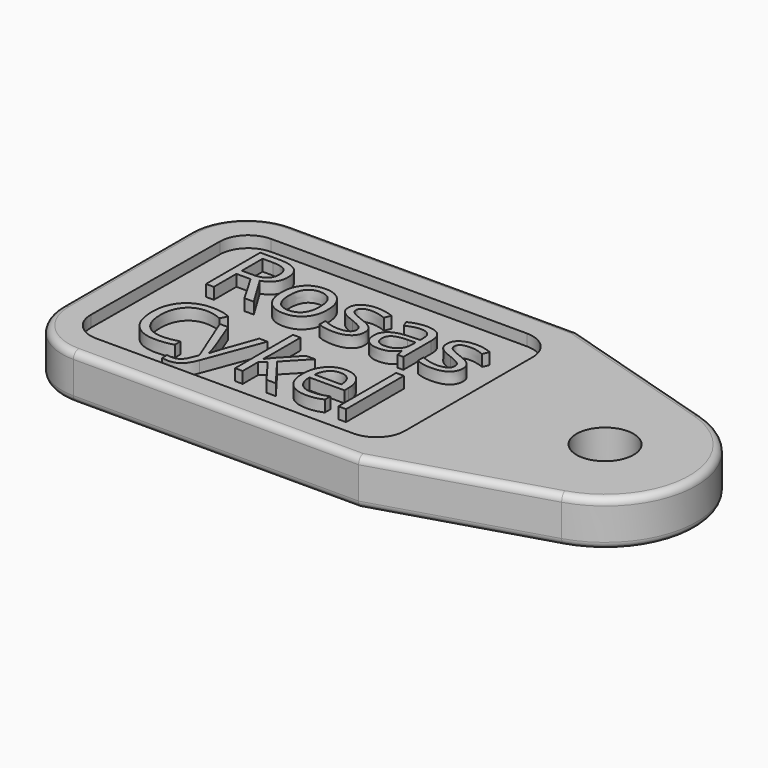
from build123d import *

# Parameters (mm, degrees)
F1_DEPTH     = 3
F2_TEXT_SIZE = 8.3333333333
F3_DEPTH     = 1
F4_R         = 0.6
F5_DEPTH     = 1
F6_D         = 5
F7_R         = 0.6


# Not quite as in the source:
# - Text() gives the source's letters only with a copy of the font that has no kerning and outlines rounded to 1/6400 em; it was checked with that copy


with BuildPart() as f1:
    # F0 (on Top) → F1 (new body)
    with BuildSketch(Plane.XY):
        with BuildLine():
            Line((30, 12), (5, 12))
            ThreePointArc((5, 12), (1.4644660941, 10.5355339059), (0, 7))
            Line((0, 7), (0, -7))
            ThreePointArc((0, -7), (1.4644660941, -10.5355339059), (5, -12))
            Line((5, -12), (30, -12))
            Line((30, -12), (44.322209849, -7.6555431824))
            ThreePointArc((44.322209849, -7.6555431824), (50, 0), (44.322209849, 7.6555431824))
            Line((44.322209849, 7.6555431824), (30, 12))
        make_face()
    extrude(amount=F1_DEPTH)

    # F2 (on face) → F3 (join)
    with BuildSketch(Plane.XY.offset(3)):
        with Locations((5, 1.5)):
            Text('Rosas', F2_TEXT_SIZE, font='Open Sans', text_align=(TextAlign.LEFT, TextAlign.BOTTOM))
        with Locations((5, -7)):
            Text('Cykel', F2_TEXT_SIZE, font='Open Sans', text_align=(TextAlign.LEFT, TextAlign.BOTTOM))
    extrude(amount=F3_DEPTH)

    # F4
    f4_edges = [f1.edges().sort_by_distance(p)[0] for p in [
        (1.464466, -10.535534, 0),
        (37.161105, -9.827772, 0),
    ]]
    fillet(f4_edges, radius=F4_R)

    # F2 (on face) → F5 (join)
    with BuildSketch(Plane.XY.offset(3)):
        with BuildLine():
            ThreePointArc((44.322209849, -7.6555431824), (50, 0), (44.322209849, 7.6555431824))
            Line((44.322209849, 7.6555431824), (30, 12))
            Line((30, 12), (5, 12))
            ThreePointArc((5, 12), (1.4644660941, 10.5355339059), (0, 7))
            Line((0, 7), (0, -7))
            ThreePointArc((0, -7), (1.4644660941, -10.5355339059), (5, -12))
            Line((5, -12), (30, -12))
            Line((30, -12), (44.322209849, -7.6555431824))
        make_face()
        with BuildLine():
            ThreePointArc((2.6266098272, 7.0191604938), (3.3655567355, 8.7745282802), (5.1265364012, 9.5))
            Line((5.1265364012, 9.5), (27.5572421402, 9.5))
            ThreePointArc((27.5572421402, 9.5), (29.3250090931, 8.767766953), (30.0572421402, 7))
            Line((30.0572421402, 7), (30.0572421402, -7))
            ThreePointArc((30.0572421402, -7), (29.3250090931, -8.767766953), (27.5572421402, -9.5))
            Line((27.5572421402, -9.5), (5.0192344847, -9.5))
            ThreePointArc((5.0192344847, -9.5), (3.2447062045, -8.7609796656), (2.5193079106, -6.9808395062))
            Line((2.5193079106, -6.9808395062), (2.6266098272, 7.0191604938))
        make_face(mode=Mode.SUBTRACT)
    extrude(amount=F5_DEPTH)

    # F6 (through all)
    with Locations(Plane(origin=(0, 0, 0), x_dir=(1, 0, 0), z_dir=(0, 0, -1))):
        with Locations((42, 0)):
            Hole(F6_D / 2)

    # F7
    f7_edges = [f1.edges().sort_by_distance(p)[0] for p in [
        (17.5, 12, 4),
        (37.161105, 9.827772, 4),
    ]]
    fillet(f7_edges, radius=F7_R)


solid = f1.part
